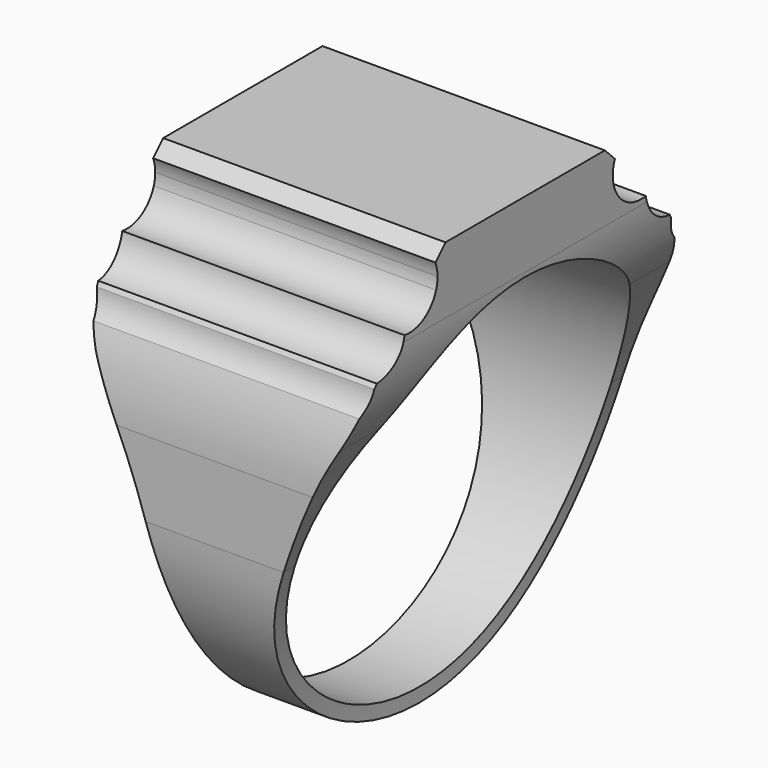
from build123d import *

# Parameters (mm, degrees)
F0_R      = 14
F1_DEPTH  = 20
F2_SIZE   = 10
F4_DEPTH  = 38.6586394161
F5_R      = 13.8386431078
F6_F1_R   = 12
F6_F2_R   = 12
F7_W      = 49.8866699636
F7_H      = 41.0156846046
F8_DEPTH  = 38.5990254581
F10_DEPTH = 25


with BuildPart() as f1:
    # F0 (on Right) → F1 (new body)
    with BuildSketch(Plane.YZ):
        with BuildLine():
            Line((-15, 21.0786387324), (-15, 0))
            ThreePointArc((-15, 0), (0, -15), (15, 0))
            Line((15, 0), (15, 21.0786387324))
            Line((15, 21.0786387324), (-15, 21.0786387324))
        make_face()
        Circle(F0_R, mode=Mode.SUBTRACT)
    extrude(amount=F1_DEPTH)

    # F2
    f2_edges = [f1.edges().sort_by_distance(p)[0] for p in [
        (10, -15, 21.078639),
        (10, 15, 21.078639),
    ]]
    chamfer(f2_edges, length=F2_SIZE)

    # F3 (on face) → F4 (cut)
    with BuildSketch(Plane(origin=(0, 15, 0), x_dir=(-1, 0, 0), z_dir=(0, 1, 0))):
        with BuildLine():
            Line((-5.1145853621, 0), (0, 0))
            Line((0, 0), (0, 11.0786387324))
            ThreePointArc((0, 11.0786387324), (-2.8965213104, 5.6959282984), (-5.1145853621, 0))
        make_face()
        with BuildLine():
            Line((-20, 0), (-14.8854146379, 0))
            ThreePointArc((-14.8854146379, 0), (-17.1034786896, 5.6959282984), (-20, 11.0786387324))
            Line((-20, 11.0786387324), (-20, 0))
        make_face()
        with BuildLine():
            Line((-20, -15), (-12.5, -15))
            ThreePointArc((-12.5, -15), (-13.1198156851, -7.4088943941), (-14.8854146379, 0))
            Line((-14.8854146379, 0), (-20, 0))
            Line((-20, 0), (-20, -15))
        make_face()
        with BuildLine():
            Line((-7.5, -15), (0, -15))
            Line((0, -15), (0, 0))
            Line((0, 0), (-5.1145853621, 0))
            ThreePointArc((-5.1145853621, 0), (-6.8801843149, -7.4088943941), (-7.5, -15))
        make_face()
    extrude(amount=-F4_DEPTH, mode=Mode.SUBTRACT)

    # F5
    f5_edges = [f1.edges().sort_by_distance(p)[0] for p in [
        (10, 15, 11.078639),
        (10, -15, 11.078639),
    ]]
    fillet(f5_edges, radius=F5_R)

    # F6: fillet of radius 12 on 4 edges, made by hand

    # F6_f1
    f6_f1_edges = [f1.edges().sort_by_distance(p)[0] for p in [
        (0, -11.1582173276, 11.0786387324),
    ]]
    fillet(f6_f1_edges, radius=F6_F1_R)

    # F6_f2
    f6_f2_edges = [f1.edges().sort_by_distance(p)[0] for p in [
        (20, -11.1582173276, 11.0786387324),
    ]]
    fillet(f6_f2_edges, radius=F6_F2_R)

    # F7 (on Right) → F8 (cut, symmetric)
    with BuildSketch(Plane.YZ):
        with Locations((-1.9184369594, 39.5302809775)):
            Rectangle(F7_W, F7_H)
    extrude(amount=F8_DEPTH, both=True, mode=Mode.SUBTRACT)

    # F9 (on Right) → F10 (cut)
    with BuildSketch(Plane.YZ):
        with BuildLine():
            ThreePointArc((13.1383126183, 12.5615130593), (13.6820509432, 10.9110715325), (15.1701192952, 10.0137080727))
            ThreePointArc((15.1701192952, 10.0137080727), (15.5705478949, 10.9205773773), (16.2919620049, 11.6005161105))
            ThreePointArc((16.2919620049, 11.6005161105), (15.6366296494, 12.4697960372), (14.9349695532, 13.3021308235))
            ThreePointArc((14.9349695532, 13.3021308235), (14.111548562, 12.7501046734), (13.1383126183, 12.5615130593))
        make_face()
        with BuildLine():
            ThreePointArc((10.6842297635, 14.7055806807), (11.5139277039, 13.1787506551), (13.1383126183, 12.5615130593))
            ThreePointArc((13.1383126183, 12.5615130593), (13.3703783986, 13.5253078885), (13.9587913382, 14.3231331899))
            ThreePointArc((13.9587913382, 14.3231331899), (13.1587745188, 15.0614293201), (12.3197712741, 15.755101896))
            ThreePointArc((12.3197712741, 15.755101896), (11.6081510723, 15.0649195379), (10.6842297635, 14.7055806807))
        make_face()
        with BuildLine():
            ThreePointArc((11.1769736326, 16.5853929835), (10.7404739393, 15.6953238755), (10.6842297635, 14.7055806807))
            ThreePointArc((10.6842297635, 14.7055806807), (11.6081510723, 15.0649195379), (12.3197712741, 15.755101896))
            ThreePointArc((12.3197712741, 15.755101896), (11.7557050458, 16.1803398875), (11.1769736326, 16.5853929835))
        make_face()
        with BuildLine():
            ThreePointArc((7.8867469732, 16.3769988391), (8.9757373546, 15.022853888), (10.6842297635, 14.7055806807))
            ThreePointArc((10.6842297635, 14.7055806807), (10.7404739393, 15.6953238755), (11.1769736326, 16.5853929835))
            ThreePointArc((11.1769736326, 16.5853929835), (10.2579855481, 17.168975872), (9.3086054096, 17.7016910302))
            ThreePointArc((9.3086054096, 17.7016910302), (8.7316580559, 16.895535493), (7.8867469732, 16.3769988391))
        make_face()
        with BuildLine():
            ThreePointArc((8.0359187979, 18.3145846001), (7.7653618104, 17.3608792391), (7.8867469732, 16.3769988391))
            ThreePointArc((7.8867469732, 16.3769988391), (8.7316580559, 16.895535493), (9.3086054096, 17.7016910302))
            ThreePointArc((9.3086054096, 17.7016910302), (8.6776747824, 18.019377358), (8.0359187979, 18.3145846001))
        make_face()
        with BuildLine():
            ThreePointArc((-9.3086054096, 17.7016910302), (-8.7316580559, 16.895535493), (-7.8867469732, 16.3769988391))
            ThreePointArc((-7.8867469732, 16.3769988391), (-7.7903858604, 16.7677879095), (-7.7579855481, 17.168975872))
            ThreePointArc((-7.7579855481, 17.168975872), (-7.8284622538, 17.758396403), (-8.0359187979, 18.3145846001))
            ThreePointArc((-8.0359187979, 18.3145846001), (-8.6776747824, 18.019377358), (-9.3086054096, 17.7016910302))
        make_face()
        with BuildLine():
            ThreePointArc((-10.6842297635, 14.7055806807), (-8.9757373546, 15.022853888), (-7.8867469732, 16.3769988391))
            ThreePointArc((-7.8867469732, 16.3769988391), (-8.7316580559, 16.895535493), (-9.3086054096, 17.7016910302))
            ThreePointArc((-9.3086054096, 17.7016910302), (-10.2579855481, 17.168975872), (-11.1769736326, 16.5853929835))
            ThreePointArc((-11.1769736326, 16.5853929835), (-10.79186702, 15.8662578063), (-10.6587745188, 15.0614293201))
            ThreePointArc((-10.6587745188, 15.0614293201), (-10.6651464503, 14.883050353), (-10.6842297635, 14.7055806807))
        make_face()
        with BuildLine():
            ThreePointArc((-12.3197712741, 15.755101896), (-11.6081510723, 15.0649195379), (-10.6842297635, 14.7055806807))
            ThreePointArc((-10.6842297635, 14.7055806807), (-10.6651464503, 14.883050353), (-10.6587745188, 15.0614293201))
            ThreePointArc((-10.6587745188, 15.0614293201), (-10.79186702, 15.8662578063), (-11.1769736326, 16.5853929835))
            ThreePointArc((-11.1769736326, 16.5853929835), (-11.7557050458, 16.1803398875), (-12.3197712741, 15.755101896))
        make_face()
        with BuildLine():
            ThreePointArc((-13.1383126183, 12.5615130593), (-11.5139277039, 13.1787506551), (-10.6842297635, 14.7055806807))
            ThreePointArc((-10.6842297635, 14.7055806807), (-11.6081510723, 15.0649195379), (-12.3197712741, 15.755101896))
            ThreePointArc((-12.3197712741, 15.755101896), (-13.1587745188, 15.0614293201), (-13.9587913382, 14.3231331899))
            ThreePointArc((-13.9587913382, 14.3231331899), (-13.3703783986, 13.5253078885), (-13.1383126183, 12.5615130593))
        make_face()
        with BuildLine():
            ThreePointArc((-13.1366296494, 12.4697960372), (-13.137050427, 12.5156622681), (-13.1383126183, 12.5615130593))
            ThreePointArc((-13.1383126183, 12.5615130593), (-14.111548562, 12.7501046734), (-14.9349695532, 13.3021308235))
            ThreePointArc((-14.9349695532, 13.3021308235), (-15.6366296494, 12.4697960372), (-16.2919620049, 11.6005161105))
            ThreePointArc((-16.2919620049, 11.6005161105), (-15.5705478949, 10.9205773773), (-15.1701192952, 10.0137080727))
            ThreePointArc((-15.1701192952, 10.0137080727), (-13.7109770476, 10.8754742198), (-13.1366296494, 12.4697960372))
        make_face()
    extrude(amount=F10_DEPTH, mode=Mode.SUBTRACT)


solid = f1.part
